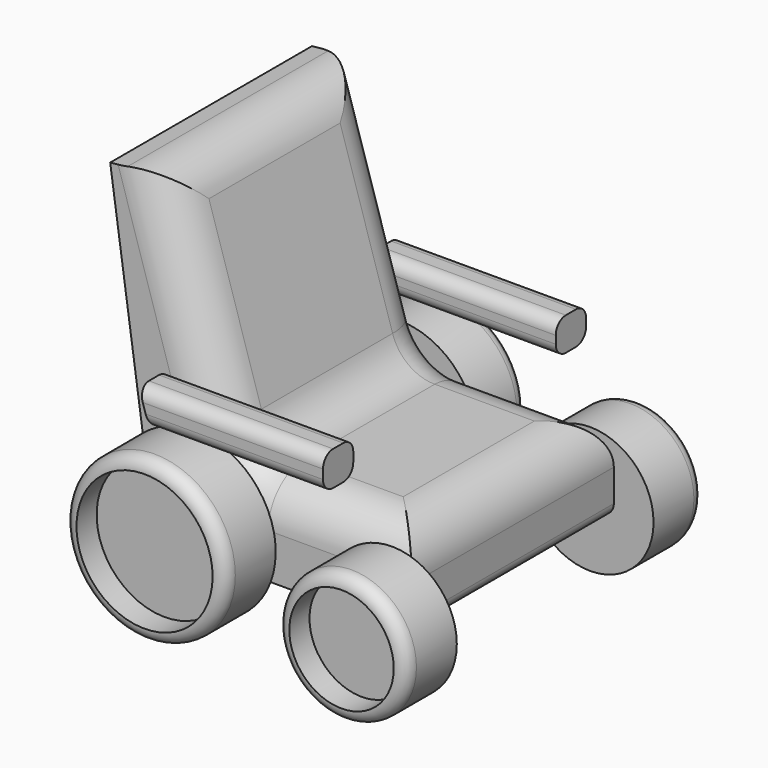
from build123d import *

# Parameters (mm, degrees)
F1_DEPTH  = 101.6
F2_F1_R   = 17.78
F2_F2_R   = 17.78
F3_R      = 25.5257149729
F3_R_2    = 30.9932269238
F4_DEPTH  = 25.4
F5_R      = 32.4962877328
F5_R_2    = 26.1094641949
F6_DEPTH  = 25.4
F8_DEPTH  = 15.24
F9_R      = 5.08
F11_DEPTH = 15.24
F12_R     = 5.08
F12_2_R   = 5.08
F13_R     = 5.08
F14_DEPTH = 10.16
F15_DEPTH = 10.16
F16_DEPTH = 10.16


with BuildPart() as f1:
    # F0 (on Front) → F1 (new body)
    with BuildSketch(Plane.XZ):
        Polygon((-12.505765073, -18.4224713594), (-41.8203547597, 75.7069438696), (-63.0667060614, 73.5554099083), (-44.7787046432, -54.1916489601), (58.4947057068, -54.1916489601), (58.4947057068, -18.4224713594), align=None)
    extrude(amount=F1_DEPTH)

    # F2: fillet of radius 17.78 on 5 edges, made by hand

    # F2_f1
    f2_f1_edges = [f1.edges().sort_by_distance(p)[0] for p in [
        (-12.505765073, -50.8, -18.4224713594),
    ]]
    fillet(f2_f1_edges, radius=F2_F1_R)

    # F2_f2
    f2_f2_edges = [f1.edges().sort_by_distance(p)[0] for p in [
        (29.5370058814, -101.6, -18.4224713594),
        (29.5370058814, 0, -18.4224713594),
        (58.4947057068, -50.8, -18.4224713594),
        (-41.8203547597, -50.8, 75.7069438696),
        (-9.9594288223, 0, -14.9625086208),
        (-9.9594288223, -101.6, -14.9625086208),
    ]]
    fillet(f2_f2_edges, radius=F2_F2_R)

    # F3 (on Front) → F4 (join)
    with BuildSketch(Plane.XZ):
        with Locations((48.9659570158, -50.5978167057)):
            Circle(F3_R)
        with Locations((-27.7856793255, -43.291490525)):
            Circle(F3_R_2)
    extrude(amount=-F4_DEPTH)

    # F5 (on face) → F6 (join)
    with BuildSketch(Plane.XZ.offset(101.6)):
        with Locations((-28.9111752063, -42.8961217403)):
            Circle(F5_R)
        with Locations((50.4264719784, -51.7711788416)):
            Circle(F5_R_2)
    extrude(amount=F6_DEPTH)

    # F13
    f13_edges = [f1.edges().sort_by_distance(p)[0] for p in [
        (-61.407463, -127, -42.896122),
        (24.317008, -127, -51.771179),
        (23.440242, 25.4, -50.597817),
        (-58.778906, 25.4, -43.291491),
        (58.494706, -50.8, -54.191649),
    ]]
    fillet(f13_edges, radius=F13_R)

    # F14 (cut): a face of the model
    f14_faces = [f1.faces().sort_by_distance(p)[0] for p in [
        (50.4264719784, -127, -51.7711788416),
    ]]
    extrude(f14_faces, amount=-F14_DEPTH, mode=Mode.SUBTRACT)

    # F15 (cut): faces of the model
    f15_faces = [f1.faces().sort_by_distance(p)[0] for p in [
        (48.9659570158, 25.4, -50.5978167057),
        (-27.7856793255, 25.4, -43.291490525),
    ]]
    extrude(f15_faces, amount=-F15_DEPTH, mode=Mode.SUBTRACT)

    # F16 (cut): a face of the model
    f16_faces = [f1.faces().sort_by_distance(p)[0] for p in [
        (-28.9111752063, -127, -42.8961217403),
    ]]
    extrude(f16_faces, amount=-F16_DEPTH, mode=Mode.SUBTRACT)


with BuildPart() as f8:
    # F7 (on face) → F8 (new body)
    with BuildSketch(Plane.XZ.offset(101.6)):
        Polygon((34.8361097276, 7.9966569319), (-39.355707759, 7.9966569319), (-35.0370473262, -5.8706011623), (34.8361097276, -5.8706011623), align=None)
    extrude(amount=F8_DEPTH)

    # F9
    f9_edges = [f8.edges().sort_by_distance(p)[0] for p in [
        (-2.259799, -116.84, 7.996657),
        (-0.100469, -116.84, -5.870601),
        (-2.259799, -101.6, 7.996657),
    ]]
    fillet(f9_edges, radius=F9_R)

    # F12#2
    f12_2_edges = [f8.edges().sort_by_distance(p)[0] for p in [
        (-0.100469, -101.6, -5.870601),
    ]]
    fillet(f12_2_edges, radius=F12_2_R)


with BuildPart() as f11:
    # F10 (on face) → F11 (new body)
    with BuildSketch(Plane(origin=(0, 0, 0), x_dir=(-1, 0, 0), z_dir=(0, 1, 0))):
        Polygon((39.355707759, 7.9966569319), (-35.1080186665, 7.9966569319), (-35.1080186665, -5.3267870098), (35.206406593, -5.3267870098), align=None)
    extrude(amount=F11_DEPTH)

    # F12
    f12_edges = [f11.edges().sort_by_distance(p)[0] for p in [
        (-2.123845, 15.24, 7.996657),
        (-2.123845, 0, 7.996657),
        (-0.049194, 15.24, -5.326787),
        (-0.049194, 0, -5.326787),
    ]]
    fillet(f12_edges, radius=F12_R)


solid = Compound([f1.part, f8.part, f11.part])
